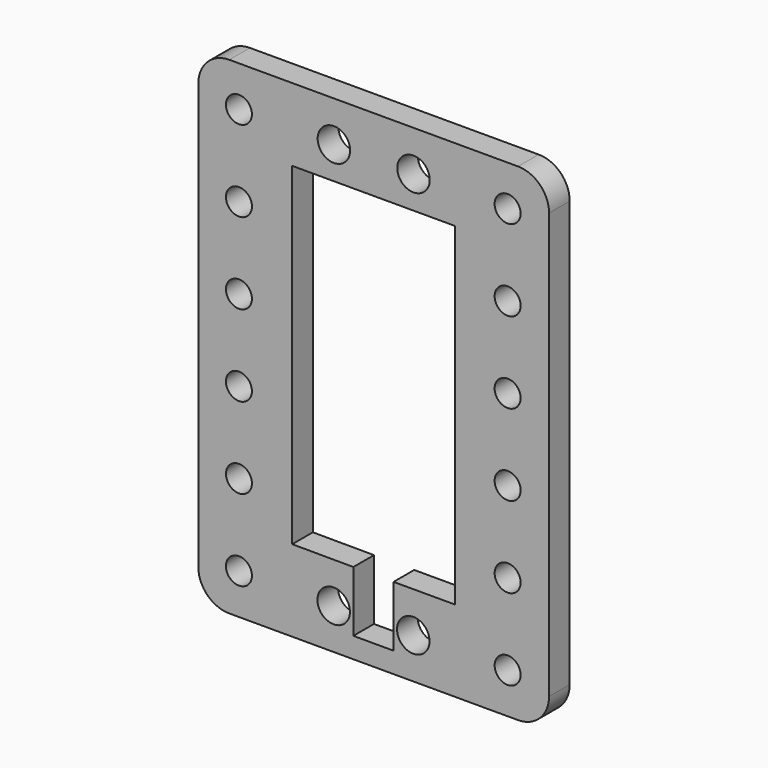
from build123d import *

# Parameters (mm, degrees)
F0_R     = 1.6
F0_R_2   = 2
F1_DEPTH = 3.175


# Not quite as in the source:
# - a length typed as a fraction of an inch, garbled in the dataset ("3 / 203.2 mm" for 3/8 in), is restored


with BuildPart() as f1:
    # F0 (on Front) → F1 (new body)
    with BuildSketch(Plane.XZ):
        with BuildLine():
            Line((27.8025, 8.975), (-7.7525, 8.975))
            ThreePointArc((-7.7525, 8.975), (-10.4465768363, 7.8590768363), (-11.5625, 5.165))
            Line((-11.5625, 5.165), (-11.5625, -47.215))
            ThreePointArc((-11.5625, -47.215), (-10.4465768363, -49.9090768363), (-7.7525, -51.025))
            Line((-7.7525, -51.025), (27.8025, -51.025))
            ThreePointArc((27.8025, -51.025), (30.4965768363, -49.9090768363), (31.6125, -47.215))
            Line((31.6125, -47.215), (31.6125, 5.165))
            ThreePointArc((31.6125, 5.165), (30.4965768363, 7.8590768363), (27.8025, 8.975))
        make_face()
        with Locations((-6.5625, -46.025)):
            Circle(F0_R, mode=Mode.SUBTRACT)
        with Locations((5.1, -46.025)):
            Circle(F0_R_2, mode=Mode.SUBTRACT)
        with Locations((-6.5625, -36.025)):
            Circle(F0_R, mode=Mode.SUBTRACT)
        with Locations((-6.5625, -26.025)):
            Circle(F0_R, mode=Mode.SUBTRACT)
        Polygon((0, -41), (0, 0), (20.025, 0), (20.025, -41.025), (12.4728614733, -41.025), (12.4728614733, -48.485), (7.5228614733, -48.485), (7.5228614733, -41.025), align=None, mode=Mode.SUBTRACT)
        with Locations((14.9, -46.025)):
            Circle(F0_R_2, mode=Mode.SUBTRACT)
        with Locations((26.5125, -46.025)):
            Circle(F0_R, mode=Mode.SUBTRACT)
        with Locations((26.5125, -36.025)):
            Circle(F0_R, mode=Mode.SUBTRACT)
        with Locations((26.5125, -26.025)):
            Circle(F0_R, mode=Mode.SUBTRACT)
        with Locations((-6.5625, -16.025)):
            Circle(F0_R, mode=Mode.SUBTRACT)
        with Locations((-6.5625, -6.025)):
            Circle(F0_R, mode=Mode.SUBTRACT)
        with Locations((-6.5625, 3.975)):
            Circle(F0_R, mode=Mode.SUBTRACT)
        with Locations((5.125, 3.975)):
            Circle(F0_R_2, mode=Mode.SUBTRACT)
        with Locations((26.5125, -16.025)):
            Circle(F0_R, mode=Mode.SUBTRACT)
        with Locations((14.925, 3.975)):
            Circle(F0_R_2, mode=Mode.SUBTRACT)
        with Locations((26.5125, -6.025)):
            Circle(F0_R, mode=Mode.SUBTRACT)
        with Locations((26.5125, 3.975)):
            Circle(F0_R, mode=Mode.SUBTRACT)
    extrude(amount=F1_DEPTH)


solid = f1.part
